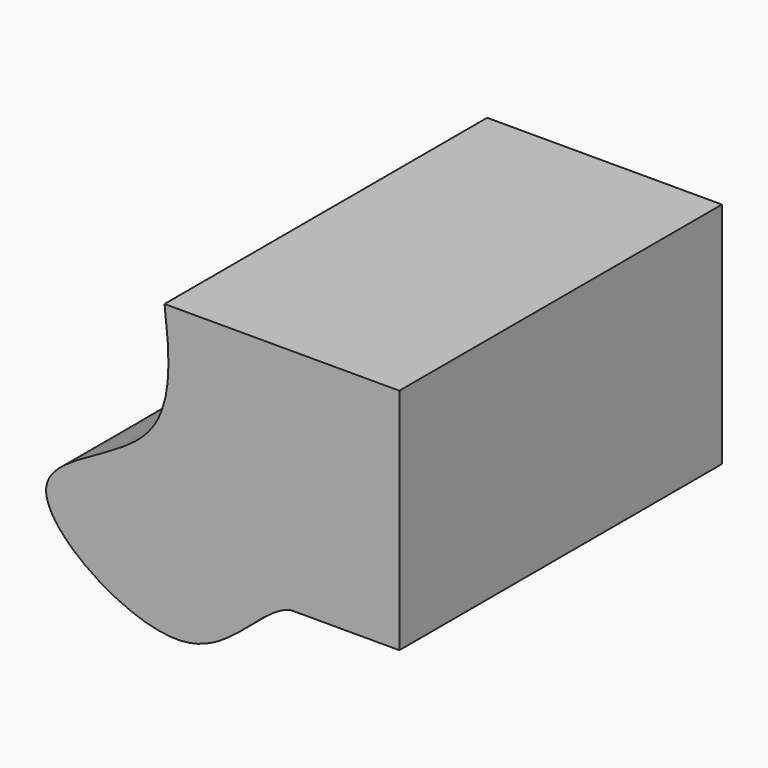
from build123d import *

# Parameters (mm, degrees)
F1_W     = 76.2
F1_H     = 76.2
F2_DEPTH = 76.2
F4_DEPTH = 76.2


# Not quite as in the source:
# - a variable given as a bare number and used for a length is read in inches; the dataset says mm whatever the document's units were


with BuildPart() as f2:
    # F1 (on Front) → F2 (new body)
    with BuildSketch(Plane.XZ):
        Rectangle(F1_W, F1_H)
    extrude(amount=F2_DEPTH)

    # F3 (on face) → F4 (cut)
    with BuildSketch(Plane.XZ.offset(76.2)):
        with BuildLine():
            add(Edge.make_bspline(
                [(-6.2764575705, 38.1), (-5.3221160752, 29.749324156), (-3.3015376501, 12.0652499196), (-42.7629516579, 2.6353877105), (0.4343283996, -27.0977029844), (11.3641512474, -6.7613463281), (17.4378827214, -5.08)],
                knots=[0, 0, 0, 0, 0.2399972153, 0.4832807981, 0.7593961967, 1, 1, 1, 1], degree=3))
            Line((-6.2764575705, 38.1), (-38.1, 38.1))
            Line((-38.1, 38.1), (-38.1, -38.1))
            Line((-38.1, -38.1), (38.1, -38.1))
            Line((38.1, -38.1), (38.1, -5.08))
            Line((38.1, -5.08), (17.4378827214, -5.08))
        make_face()
    extrude(amount=-F4_DEPTH, mode=Mode.SUBTRACT)


solid = f2.part
